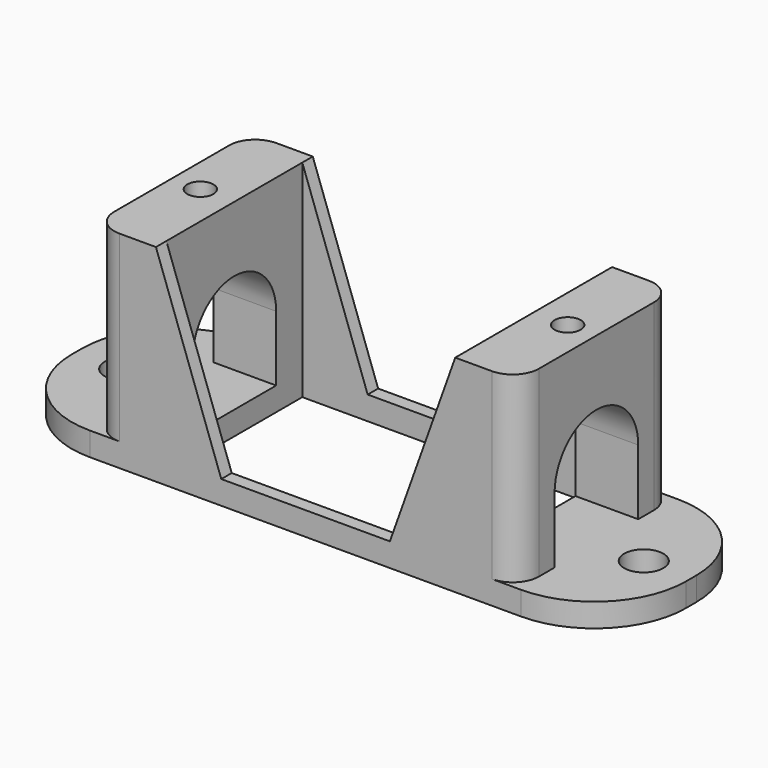
from build123d import *

# Parameters (mm, degrees)
F0_W      = 47
F0_H      = 15
F1_DEPTH  = 1.8
F3_DEPTH  = 14
F4_W      = 22.9
F4_H      = 13
F5_DEPTH  = 15.801
F6_R      = 1
F7_DEPTH  = 7
F8_R      = 1.5
F9_R      = 1.5
F10_DEPTH = 1.801
F12_DEPTH = 39.751
F13_R     = 7
F15_DEPTH = 1.001
F16_DEPTH = 14.001
F17_R     = 2


with BuildPart() as f1:
    # F0 (on Top) → F1 (new body)
    with BuildSketch(Plane.XY):
        with Locations((23.5, 7.5)):
            Rectangle(F0_W, F0_H)
    extrude(amount=F1_DEPTH)

    # F2 (on face) → F3 (join)
    with BuildSketch(Plane.XY.offset(1.8)):
        Polygon((39.75, 15), (23.5, 15), (7.25, 15), (7.25, 0), (23.5, 0), (39.75, 0), align=None)
    extrude(amount=F3_DEPTH)

    # F4 (on face) → F5 (cut, through all)
    with BuildSketch(Plane.XY.offset(15.8)):
        with Locations((23.5, 7.5)):
            Rectangle(F4_W, F4_H)
    extrude(amount=-F5_DEPTH, mode=Mode.SUBTRACT)

    # F6 (on face) → F7 (cut)
    with BuildSketch(Plane.XY.offset(15.8)):
        with Locations((9.45, 7.5)):
            Circle(F6_R)
        with Locations((37.55, 7.5)):
            Circle(F6_R)
    extrude(amount=-F7_DEPTH, mode=Mode.SUBTRACT)

    # F8 (on face) + F9 (on face) → F10 (cut, through all)
    with BuildSketch(Plane.XY.offset(1.8)):
        with Locations((3.625, 7.5)):
            Circle(F8_R)
    with BuildSketch(Plane.XY.offset(1.8)):
        with Locations((43.375, 7.5)):
            Circle(F9_R)
    extrude(amount=-F10_DEPTH, mode=Mode.SUBTRACT)

    # F11 (on face) → F12 (cut, through all)
    with BuildSketch(Plane(origin=(7.25, 0, 0), x_dir=(0, -1, 0), z_dir=(-1, 0, 0))):
        with BuildLine():
            Line((-11.5, 1.8), (-3.5, 1.8))
            Line((-3.5, 1.8), (-3.5, 6.8))
            ThreePointArc((-3.5, 6.8), (-7.5, 10.8), (-11.5, 6.8))
            Line((-11.5, 6.8), (-11.5, 1.8))
        make_face()
    extrude(amount=-F12_DEPTH, mode=Mode.SUBTRACT)

    # F13
    f13_edges = [f1.edges().sort_by_distance(p)[0] for p in [
        (0, 15, 0.9),
        (0, 0, 0.9),
        (47, 0, 0.9),
        (47, 15, 0.9),
    ]]
    fillet(f13_edges, radius=F13_R)

    # F14 (on face) → F15 (cut, through all)
    with BuildSketch(Plane.XZ.offset(-14)):
        Polygon((34.95, 15.8), (12.05, 15.8), (17.05, 1.8), (29.95, 1.8), align=None)
    extrude(amount=-F15_DEPTH, mode=Mode.SUBTRACT)

    # F14 (on face) → F16 (cut, through all)
    with BuildSketch(Plane.XZ.offset(-14)):
        Polygon((34.95, 15.8), (12.05, 15.8), (17.05, 1.8), (29.95, 1.8), align=None)
    extrude(amount=F16_DEPTH, mode=Mode.SUBTRACT)

    # F17
    f17_edges = [f1.edges().sort_by_distance(p)[0] for p in [
        (39.75, 15, 8.8),
        (39.75, 0, 8.8),
        (7.25, 0, 8.8),
        (7.25, 15, 8.8),
    ]]
    fillet(f17_edges, radius=F17_R)


solid = f1.part
